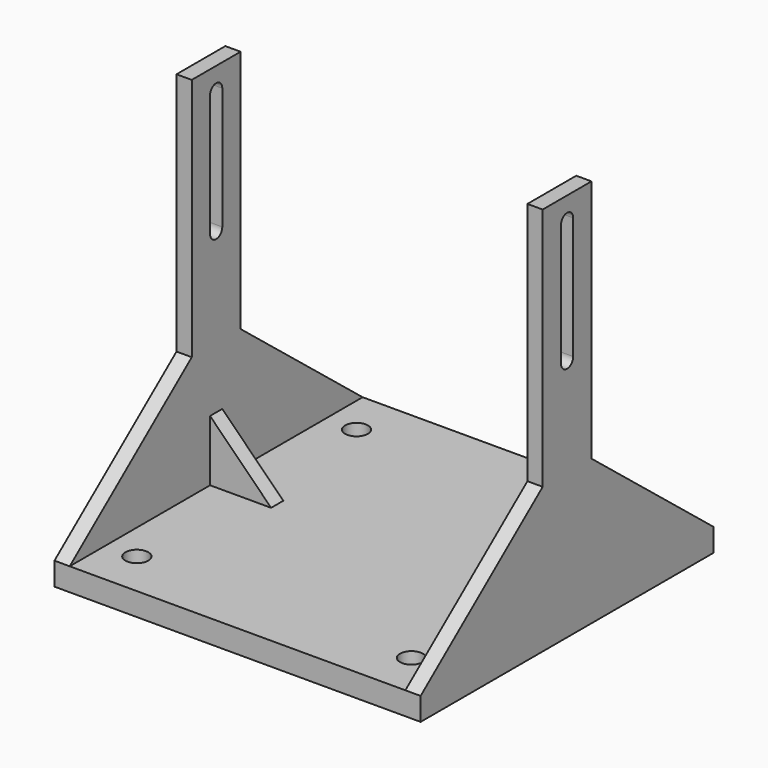
from build123d import *

# Parameters (mm, degrees)
F0_W      = 304.8
F0_H      = 304.8
F1_DEPTH  = 19.05
F2_W      = 12.7
F2_H      = 50.8
F3_DEPTH  = 304.8
F5_DEPTH  = 25.4
F7_DEPTH  = 6.35
F9_DEPTH  = 12.7
F10_R     = 9.525
F11_DEPTH = 25.4


# Not quite as in the source:
# - a pattern or mirror of a feature is missing from the dataset's text; its kind, count and spacing are read off the source's solid


with BuildPart() as f1:
    # F0 (on Top) → F1 (new body)
    with BuildSketch(Plane.XY):
        Rectangle(F0_W, F0_H)
    extrude(amount=F1_DEPTH)

    # F2 (on face) → F3 (join)
    with BuildSketch(Plane.XY.offset(19.05)):
        with Locations((146.05, 0)):
            Rectangle(F2_W, F2_H)
    f3 = extrude(amount=F3_DEPTH)

    # F3_copies: F3 across plane
    add(f3.mirror(Plane(origin=(0, 0, 0), x_dir=(0, 0, -1), z_dir=(-1, 0, 0))))

    # F4 (on face) → F5 (cut)
    with BuildSketch(Plane.YZ.offset(152.4)):
        with BuildLine():
            Line((6.35, 203.2), (6.35, 304.8))
            ThreePointArc((6.35, 304.8), (0, 311.15), (-6.35, 304.8))
            Line((-6.35, 304.8), (-6.35, 203.2))
            ThreePointArc((-6.35, 203.2), (0, 196.85), (6.35, 203.2))
        make_face()
    f5 = extrude(amount=-F5_DEPTH, mode=Mode.SUBTRACT)

    # F5_copies: F5 across plane
    add(f5.mirror(Plane(origin=(0, 0, 0), x_dir=(0, 0, -1), z_dir=(-1, 0, 0))), mode=Mode.SUBTRACT)

    # F6 (on Front) → F7 (join, symmetric)
    with BuildSketch(Plane.XZ):
        Polygon((139.7, 19.05), (139.7, 69.85), (88.9, 19.05), align=None)
    f7 = extrude(amount=F7_DEPTH, both=True)

    # F7_copies: F7 across plane
    add(f7.mirror(Plane(origin=(0, 0, 0), x_dir=(0, 0, -1), z_dir=(-1, 0, 0))))

    # F8 (on face) → F9 (join)
    with BuildSketch(Plane.YZ.offset(152.4)):
        Polygon((-25.4, 120.65), (-152.4, 19.05), (-25.4, 19.05), align=None)
        Polygon((152.4, 19.05), (25.4, 120.65), (25.4, 19.05), align=None)
    f9 = extrude(amount=-F9_DEPTH)

    # F9_copies: F9 across plane
    add(f9.mirror(Plane(origin=(0, 0, 0), x_dir=(0, 0, -1), z_dir=(-1, 0, 0))))

    # F10 (on face) → F11 (cut)
    with BuildSketch(Plane.XY.offset(19.05)):
        with Locations((-114.3, 114.3)):
            Circle(F10_R)
        with Locations((114.3, 114.3)):
            Circle(F10_R)
        with Locations((114.3, -114.3)):
            Circle(F10_R)
        with Locations((-114.3, -114.3)):
            Circle(F10_R)
    extrude(amount=-F11_DEPTH, mode=Mode.SUBTRACT)


solid = f1.part
